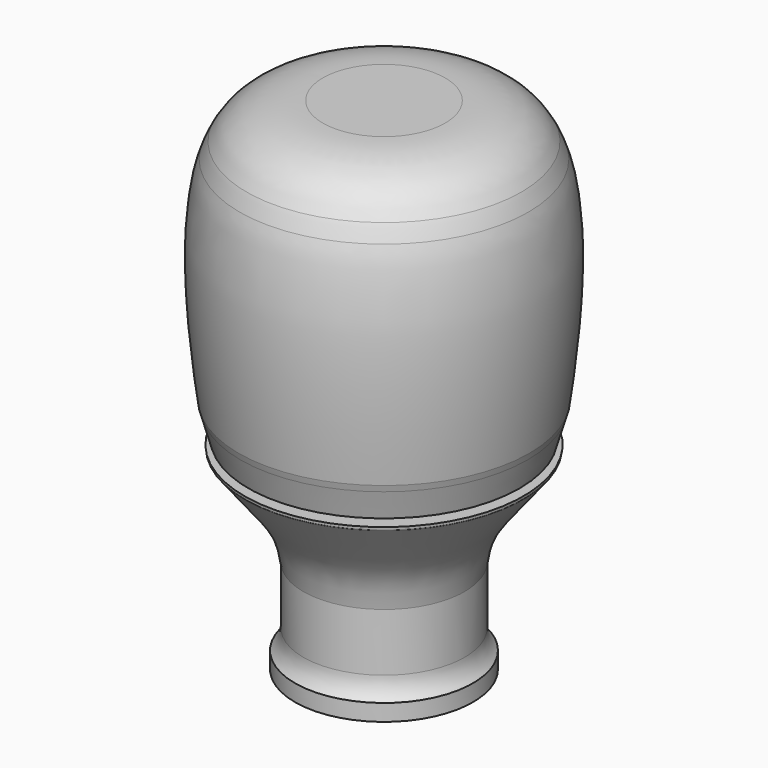
from build123d import *


# Not quite as in the source:
# - a fillet or chamfer that OpenCascade refuses, or shapes differently, is made with other operations: its cross-section is extruded or revolved along the edge and cut away or added


with BuildPart() as f1:
    # F0 (on Front) → F1 (revolve)
    with BuildSketch(Plane.XZ):
        with BuildLine():
            Line((-16, 3), (-16, 0))
            Line((-16, 0), (-11, 0))
            Line((-11, 0), (-11, 45))
            Line((-11, 45), (0, 45))
            Line((0, 45), (0, 90))
            Line((0, 90), (-11, 90))
            add(Edge.make_bspline(
                [(-11, 90), (-18.2598325737, 90), (-22.3191203043, 87.7987933146), (-24.7124240869, 83.5464183412)],
                knots=[0, 0, 0, 0, 0.3193219477, 0.3193219477, 0.3193219477, 0.3193219477], degree=3))
            add(Edge.make_bspline(
                [(-25.95214754, 80.7744236544), (-25.5955388267, 81.7789820937), (-25.1863115013, 82.7032707784), (-24.7124240769, 83.5464183618)],
                knots=[0.6173140508, 0.6173140508, 0.6173140508, 0.6173140508, 0.6804824316, 0.6804824316, 0.6804824316, 0.6804824316], degree=3))
            add(Edge.make_bspline(
                [(-25.95214754, 80.7744236544), (-29.013744824, 72.1320741786), (-28.1040669162, 57.593769762), (-25.7856152344, 41.5069436394)],
                knots=[0.3826740582, 0.3826740582, 0.3826740582, 0.3826740582, 0.9280294048, 0.9280294048, 0.9280294048, 0.9280294048], degree=3))
            Line((-25.7856152343, 41.5069436384), (-24.3623662292, 36.5477789253))
            Line((-24.3623662292, 36.5477789253), (-21.3623662292, 36.5477789253))
            Line((-21.3623662292, 36.5477789253), (-21.3623662292, 35.5477789253))
            Line((-21.3623662292, 35.5477789253), (-24.0753725342, 35.5477789253))
            Line((-24.0753725342, 35.5477789253), (-24.8771885438, 35.5477789253))
            Line((-24.8771885438, 35.5477789253), (-25.0753725342, 35.5477789253))
            add(Edge.make_bspline(
                [(-25, 35.0670883895), (-25.0252278751, 35.22739015), (-25.0503528609, 35.3876218128), (-25.0753725342, 35.5477789253)],
                knots=[0, 0, 0, 0, 0.0053759457, 0.0053759457, 0.0053759457, 0.0053759457], degree=3))
            ThreePointArc((-25, 35.0670883895), (-24.9896036739, 35.0034452685), (-24.9594955315, 34.9464186939))
            add(Edge.make_bspline(
                [(-14.5, 17), (-15.0136726081, 20.8512590653), (-16.9742007652, 25.4036532302), (-22.365796569, 31.5181893252), (-24.9594955315, 34.9464186939)],
                knots=[0, 0, 0, 0, 0.461922101, 0.9972118566, 0.9972118566, 0.9972118566, 0.9972118566], degree=3))
            Line((-14.5, 17), (-14.5, 3))
            Line((-14.5, 3), (-16, 3))
        make_face()
        with BuildLine():
            add(Edge.make_bspline(
                [(-25.95214754, 80.7744236544), (-29.013744824, 72.1320741786), (-28.1040669162, 57.593769762), (-25.7856152344, 41.5069436394)],
                knots=[0.3826740582, 0.3826740582, 0.3826740582, 0.3826740582, 0.9280294048, 0.9280294048, 0.9280294048, 0.9280294048], degree=3))
            add(Edge.make_bspline(
                [(-26.119291441, 42.669604047), (-28.2279288517, 58.1855295549), (-28.9528077457, 72.3216337444), (-25.95214754, 80.7744236544)],
                knots=[0.0857879305, 0.0857879305, 0.0857879305, 0.0857879305, 0.6173140508, 0.6173140508, 0.6173140508, 0.6173140508], degree=3))
            Line((-26.119291441, 42.669604047), (-25.7856152343, 41.5069436384))
        make_face()
    revolve(axis=Axis((0, 0, 41.293862511), (0, 0, 1)))

    # F2: fillet of radius 5.08 on 1 edges, made by hand

    # F2_s1 → F2_t2 (revolve)
    with BuildSketch(Plane.XZ):
        with BuildLine():
            ThreePointArc((-14.5, 6.6041642582), (-14.8899680172, 4.6522421286), (-16, 3))
            Line((-16, 3), (-14.5, 3))
            Line((-14.5, 3), (-14.5, 6.6041642582))
        make_face()
    revolve(axis=Axis((0, 0, 3), (0, 0, 1)))


solid = f1.part
